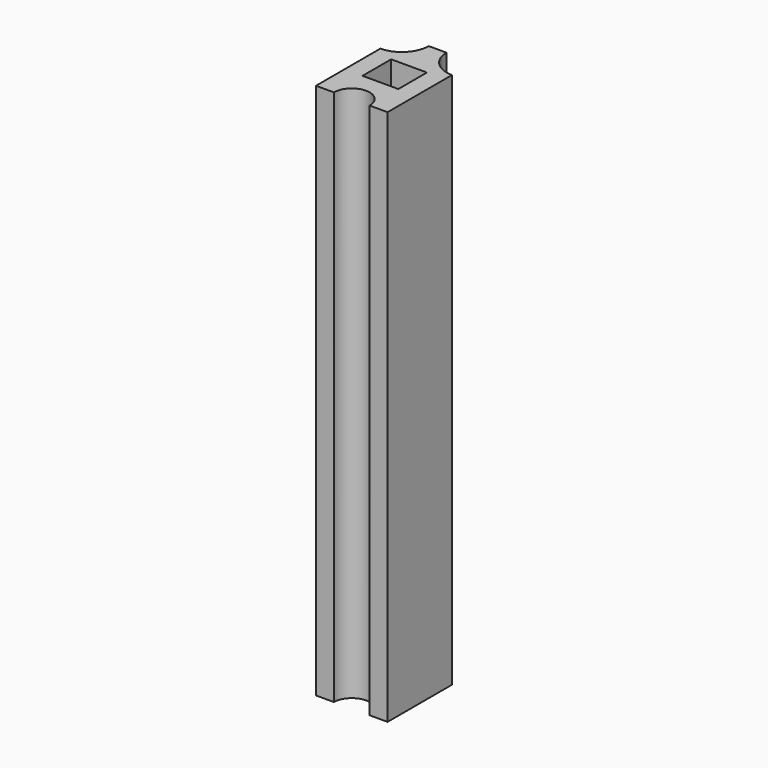
from build123d import *

# Parameters (mm, degrees)
F1_W     = 25.4
F1_H     = 25.4
F2_DEPTH = 381


# Not quite as in the source:
# - a feature of the source that left no trace in its solid (it failed there, or was rolled back) is left out


with BuildPart() as f2:
    # F1 (on Top) → F2 (new body)
    with BuildSketch(Plane.XY):
        with BuildLine():
            ThreePointArc((25.4, 19.05), (11.9296158184, 24.6296158184), (6.35, 38.1))
            Line((6.35, 38.1), (-6.35, 38.1))
            ThreePointArc((-6.35, 38.1), (-11.9296158184, 24.6296158184), (-25.4, 19.05))
            Line((-25.4, 19.05), (-25.4, -38.1))
            Line((-25.4, -38.1), (-12.7, -38.1))
            ThreePointArc((-12.7, -38.1), (0, -25.4), (12.7, -38.1))
            Line((12.7, -38.1), (25.4, -38.1))
            Line((25.4, -38.1), (25.4, 19.05))
        make_face()
        Rectangle(F1_W, F1_H, mode=Mode.SUBTRACT)
    extrude(amount=F2_DEPTH)


solid = f2.part
